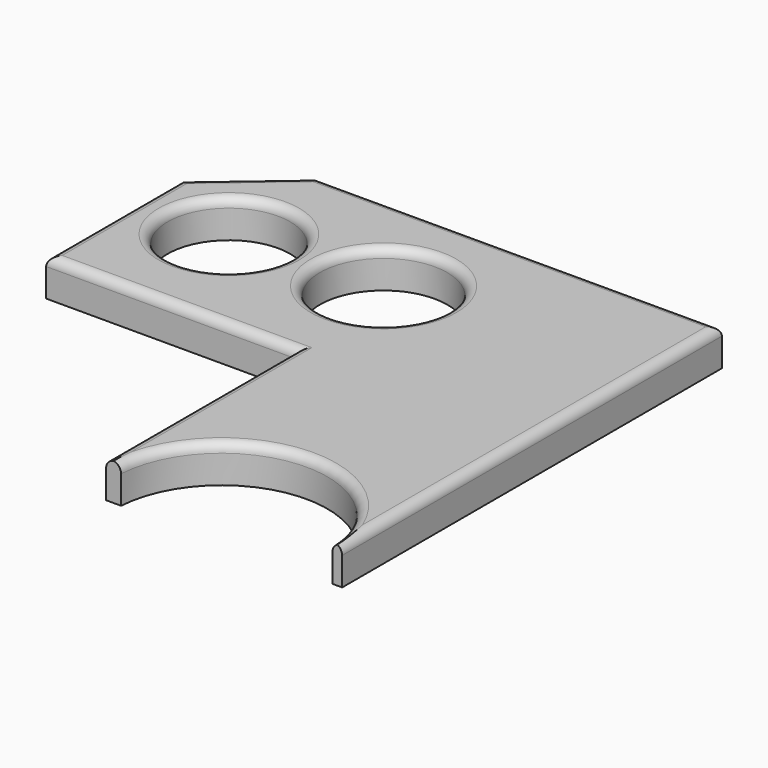
from build123d import *

# Parameters (mm, degrees)
F0_R         = 4.1761867796
F0_R_2       = 4.3460448691
F1_DEPTH     = 2.54
F2_DEPTH     = 12.7
F3_R         = 7.2200461369
F4_DEPTH     = 12.7
F7_T1_DEPTH  = 14.697191958
F7_T3_DEPTH  = 10.4099383433
F7_T5_DEPTH  = 30.8011159773
F7_T7_DEPTH  = 35.5510768625
F7_T9_DEPTH  = 17.7553157696
F7_T11_DEPTH = 18.6111496066
F7_T14_ANGLE = 198.1944914786
F7_T23_DEPTH = 17.7553157696
F7_T27_DEPTH = 18.6111496066


# Not quite as in the source:
# - a fillet or chamfer that OpenCascade refuses, or shapes differently, is made with other operations: its cross-section is extruded or revolved along the edge and cut away or added


with BuildPart() as f1:
    # F0 (on Top) → F1 (new body)
    with BuildSketch(Plane.XY):
        Polygon((-16.1636956036, 7.9843616113), (-16.1636956036, 0), (-16.1636956036, -3.5330012906), (0.857539475, -3.5330012906), (0.857539475, -6.9984025322), (16.9614627957, -6.9984025322), (16.9614627957, 0), (16.9614627957, 12.6728452742), (-10.6598241255, 12.6728452742), align=None)
        with Locations((-10.1569462568, 4.5435167849)):
            Circle(F0_R, mode=Mode.SUBTRACT)
        with Locations((0, 5.0288974307)):
            Circle(F0_R_2, mode=Mode.SUBTRACT)
    extrude(amount=F1_DEPTH)

    # F2 (add): a face of the model
    f2_faces = [f1.faces().sort_by_distance(p)[0] for p in [
        (8.9095011353, -6.9984025322, 1.27),
    ]]
    extrude(f2_faces, amount=F2_DEPTH)


with BuildPart() as f4:
    # F3 (on Top) → F4 (new body)
    with BuildSketch(Plane.XY):
        with Locations((6.5507800318, -27.7640167624)):
            Circle(F3_R)
    extrude(amount=F4_DEPTH)


with BuildPart() as f4_1:
    # F5: moved
    add(f4.part.moved(Location((2.54, 7.62, 0))))


with BuildPart() as f1_1:
    add(f1.part)

    # F6: cut F4
    add(f4_1.part, mode=Mode.SUBTRACT)

    # F7: fillet of radius 0.635 on 11 edges, made by hand

    # F7_s2 → F7_t1 (cut)
    with BuildSketch(Plane.XZ.offset(-9.5742761394)):
        with BuildLine():
            ThreePointArc((-16.1640956036, 1.9040343146), (-15.9777084097, 2.3540128061), (-15.5277299182, 2.5404))
            Line((-15.5277299182, 2.5404), (-15.5277299182, 2.6040365685))
            ThreePointArc((-15.5277299182, 2.6040365685), (-15.8457127609, 2.6036365685), (-16.1636956036, 2.6036365685))
            Line((-16.1636956036, 2.6036365685), (-16.2273321722, 2.54))
            ThreePointArc((-16.2273321722, 2.54), (-16.2273321722, 2.2220171573), (-16.2277321722, 1.9040343146))
            Line((-16.2277321722, 1.9040343146), (-16.1640956036, 1.9040343146))
        make_face()
    extrude(amount=F7_T1_DEPTH, mode=Mode.SUBTRACT)

    # F7_s4 → F7_t3 (cut)
    with BuildSketch(Plane(origin=(1.2888696755, 1.0979261491, 0), x_dir=(0, 0, 1), z_dir=(-0.7612431928, -0.6484664998, 0))):
        with BuildLine():
            ThreePointArc((1.9040343146, 16.560056038), (2.3540128061, 16.373668844), (2.5404, 15.9236903525))
            Line((2.5404, 15.9236903525), (2.6040365685, 15.9236903525))
            ThreePointArc((2.6040365685, 15.9236903525), (2.6036365685, 16.2416731952), (2.6036365685, 16.559656038))
            Line((2.6036365685, 16.559656038), (2.54, 16.6232926065))
            ThreePointArc((2.54, 16.6232926065), (2.2220171573, 16.6232926065), (1.9040343146, 16.6236926065))
            Line((1.9040343146, 16.6236926065), (1.9040343146, 16.560056038))
        make_face()
    extrude(amount=F7_T3_DEPTH, mode=Mode.SUBTRACT)

    # F7_s6 → F7_t5 (cut)
    with BuildSketch(Plane.YZ.offset(-12.2497386535)):
        with BuildLine():
            ThreePointArc((12.0368795888, 2.5404), (12.4868580803, 2.3540128061), (12.6732452742, 1.9040343146))
            Line((12.6732452742, 1.9040343146), (12.7368818428, 1.9040343146))
            ThreePointArc((12.7368818428, 1.9040343146), (12.7364818428, 2.2220171573), (12.7364818428, 2.54))
            Line((12.7364818428, 2.54), (12.6728452742, 2.6036365685))
            ThreePointArc((12.6728452742, 2.6036365685), (12.3548624315, 2.6036365685), (12.0368795888, 2.6040365685))
            Line((12.0368795888, 2.6040365685), (12.0368795888, 2.5404))
        make_face()
    extrude(amount=F7_T5_DEPTH, mode=Mode.SUBTRACT)

    # F7_s8 → F7_t7 (cut)
    with BuildSketch(Plane.XZ.offset(-14.2627598023)):
        with BuildLine():
            ThreePointArc((16.3254971103, 2.5404), (16.7754756018, 2.3540128061), (16.9618627957, 1.9040343146))
            Line((16.9618627957, 1.9040343146), (17.0254993643, 1.9040343146))
            ThreePointArc((17.0254993643, 1.9040343146), (17.0250993643, 2.2220171573), (17.0250993643, 2.54))
            Line((17.0250993643, 2.54), (16.9614627957, 2.6036365685))
            ThreePointArc((16.9614627957, 2.6036365685), (16.643479953, 2.6036365685), (16.3254971103, 2.6040365685))
            Line((16.3254971103, 2.6040365685), (16.3254971103, 2.5404))
        make_face()
    extrude(amount=F7_T7_DEPTH, mode=Mode.SUBTRACT)

    # F7_s10 → F7_t9 (cut)
    with BuildSketch(Plane.XZ.offset(3.5330012906)):
        with BuildLine():
            ThreePointArc((1.4935051604, 2.5404), (1.0435266689, 2.3540128061), (0.857139475, 1.9040343146))
            Line((0.857139475, 1.9040343146), (0.7935029064, 1.9040343146))
            ThreePointArc((0.7935029064, 1.9040343146), (0.7939029064, 2.2220171573), (0.7939029064, 2.54))
            Line((0.7939029064, 2.54), (0.857539475, 2.6036365685))
            ThreePointArc((0.857539475, 2.6036365685), (1.1755223177, 2.6036365685), (1.4935051604, 2.6040365685))
            Line((1.4935051604, 2.6040365685), (1.4935051604, 2.5404))
        make_face()
    extrude(amount=F7_T9_DEPTH, mode=Mode.SUBTRACT)

    # F7_s12 → F7_t11 (cut)
    with BuildSketch(Plane.YZ.offset(-17.7536101317)):
        with BuildLine():
            ThreePointArc((-2.8970356052, 2.5404), (-3.3470140967, 2.3540128061), (-3.5334012906, 1.9040343146))
            Line((-3.5334012906, 1.9040343146), (-3.5970378592, 1.9040343146))
            ThreePointArc((-3.5970378592, 1.9040343146), (-3.5966378592, 2.2220171573), (-3.5966378592, 2.54))
            Line((-3.5966378592, 2.54), (-3.5330012906, 2.6036365685))
            ThreePointArc((-3.5330012906, 2.6036365685), (-3.2150184479, 2.6036365685), (-2.8970356052, 2.6040365685))
            Line((-2.8970356052, 2.6040365685), (-2.8970356052, 2.5404))
        make_face()
    extrude(amount=F7_T11_DEPTH, mode=Mode.SUBTRACT)

    # F7_s13 → F7_t14 (revolve, cut)
    with BuildSketch(Plane(origin=(3.3721800717, -21.0597061225, 0), x_dir=(0, 0, 1), z_dir=(0.1581106012, -0.9874214084, 0))):
        with BuildLine():
            ThreePointArc((2.5404, 2.0645636003), (2.3540128061, 1.6145851088), (1.9040343146, 1.4281979149))
            Line((1.9040343146, 1.4281979149), (1.9040343146, 1.3645613463))
            ThreePointArc((1.9040343146, 1.3645613463), (2.2220171573, 1.3649613463), (2.54, 1.3649613463))
            Line((2.54, 1.3649613463), (2.6036365685, 1.4285979149))
            ThreePointArc((2.6036365685, 1.4285979149), (2.6036365685, 1.7465807576), (2.6040365685, 2.0645636003))
            Line((2.6040365685, 2.0645636003), (2.5404, 2.0645636003))
        make_face()
    revolve(axis=Axis((9.0907800318, -20.1440167624, 2.54), (0, 0, -1)), revolution_arc=F7_T14_ANGLE, mode=Mode.SUBTRACT)

    # F7_s15 → F7_t16 (revolve, cut)
    with BuildSketch(Plane.XZ.offset(-4.5435167849)):
        with BuildLine():
            ThreePointArc((-5.3447937917, 2.5404), (-5.7947722832, 2.3540128061), (-5.9811594771, 1.9040343146))
            Line((-5.9811594771, 1.9040343146), (-6.0447960457, 1.9040343146))
            ThreePointArc((-6.0447960457, 1.9040343146), (-6.0443960457, 2.2220171573), (-6.0443960457, 2.54))
            Line((-6.0443960457, 2.54), (-5.9807594771, 2.6036365685))
            ThreePointArc((-5.9807594771, 2.6036365685), (-5.6627766344, 2.6036365685), (-5.3447937917, 2.6040365685))
            Line((-5.3447937917, 2.6040365685), (-5.3447937917, 2.5404))
        make_face()
    revolve(axis=Axis((-10.1569462568, 4.5435167849, 2.54), (0, 0, 1)), mode=Mode.SUBTRACT)

    # F7_s17 → F7_t18 (revolve, cut)
    with BuildSketch(Plane.XZ.offset(-5.0288974307)):
        with BuildLine():
            ThreePointArc((4.9820105545, 2.5404), (4.532032063, 2.3540128061), (4.3456448691, 1.9040343146))
            Line((4.3456448691, 1.9040343146), (4.2820083005, 1.9040343146))
            ThreePointArc((4.2820083005, 1.9040343146), (4.2824083005, 2.2220171573), (4.2824083005, 2.54))
            Line((4.2824083005, 2.54), (4.3460448691, 2.6036365685))
            ThreePointArc((4.3460448691, 2.6036365685), (4.6640277118, 2.6036365685), (4.9820105545, 2.6040365685))
            Line((4.9820105545, 2.6040365685), (4.9820105545, 2.5404))
        make_face()
    revolve(axis=Axis((0, 5.0288974307, 2.54), (0, 0, 1)), mode=Mode.SUBTRACT)


with BuildPart() as f7_tool21:
    # F7_s22 → F7_t23 (new body)
    with BuildSketch(Plane.XZ.offset(1.9430867626)):
        with BuildLine():
            ThreePointArc((1.4935051604, 2.5404), (1.0435266689, 2.3540128061), (0.857139475, 1.9040343146))
            Line((0.857139475, 1.9040343146), (0.7935029064, 1.9040343146))
            ThreePointArc((0.7935029064, 1.9040343146), (0.7939029064, 2.2220171573), (0.7939029064, 2.54))
            Line((0.7939029064, 2.54), (0.857539475, 2.6036365685))
            ThreePointArc((0.857539475, 2.6036365685), (1.1755223177, 2.6036365685), (1.4935051604, 2.6040365685))
            Line((1.4935051604, 2.6040365685), (1.4935051604, 2.5404))
        make_face()
    extrude(amount=F7_T23_DEPTH)

    split(bisect_by=Plane.XZ.offset(3.5330012906), keep=Keep.BOTTOM)


with BuildPart() as f7_tool25:
    # F7_s26 → F7_t27 (new body)
    with BuildSketch(Plane.YZ.offset(-16.1636956036)):
        with BuildLine():
            ThreePointArc((-2.8970356052, 2.5404), (-3.3470140967, 2.3540128061), (-3.5334012906, 1.9040343146))
            Line((-3.5334012906, 1.9040343146), (-3.5970378592, 1.9040343146))
            ThreePointArc((-3.5970378592, 1.9040343146), (-3.5966378592, 2.2220171573), (-3.5966378592, 2.54))
            Line((-3.5966378592, 2.54), (-3.5330012906, 2.6036365685))
            ThreePointArc((-3.5330012906, 2.6036365685), (-3.2150184479, 2.6036365685), (-2.8970356052, 2.6040365685))
            Line((-2.8970356052, 2.6040365685), (-2.8970356052, 2.5404))
        make_face()
    extrude(amount=F7_T27_DEPTH)

    split(bisect_by=Plane.YZ.offset(0.857539475), keep=Keep.TOP)


with BuildPart() as f7_tool21_1:
    add(f7_tool21.part)

    # F7_t29: intersect F7_tool25
    add(f7_tool25.part, mode=Mode.INTERSECT)


with BuildPart() as f1_2:
    add(f1_1.part)

    # F7_t19: cut F7_tool21
    add(f7_tool21_1.part, mode=Mode.SUBTRACT)


solid = f1_2.part
